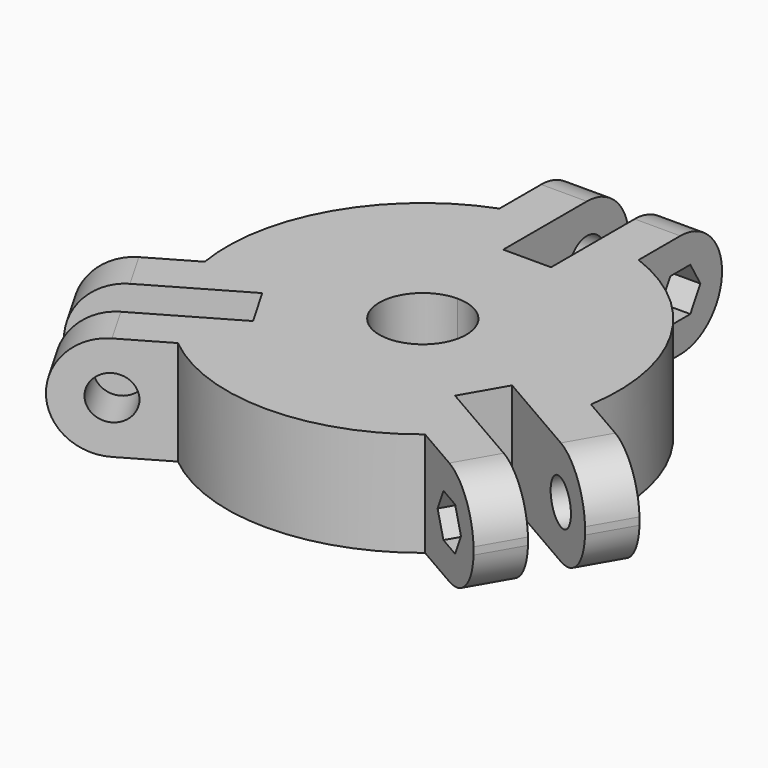
from build123d import *

# Parameters (mm, degrees)
F1_DEPTH  = 12
F3_DEPTH  = 25
F5_DEPTH  = 25
F7_DEPTH  = 25
F8_R      = 2.5
F9_DEPTH  = 5.6
F11_DEPTH = 7
F12_R     = 2.5
F13_DEPTH = 7
F15_DEPTH = 7
F16_R     = 2.5
F17_DEPTH = 7
F19_DEPTH = 7


with BuildPart() as f1:
    # F0 (on Top) → F1 (new body)
    with BuildSketch(Plane.XY):
        with BuildLine():
            ThreePointArc((0, 5), (3.5355339059, 3.5355339059), (5, 0))
            ThreePointArc((5, 0), (4.8296291314, -1.2940952255), (4.3301270189, -2.5))
            Line((4.3301270189, -2.5), (12.9903810568, -7.5))
            Line((12.9903810568, -7.5), (14.3653810568, -5.1184301396))
            Line((14.3653810568, -5.1184301396), (29.9538383249, -14.1184301396))
            Line((29.9538383249, -14.1184301396), (32.5788383249, -9.5717967697))
            Line((32.5788383249, -9.5717967697), (22.2122898066, -3.5866671921))
            ThreePointArc((22.2122898066, -3.5866671921), (19.4855715851, 11.25), (8, 21.0297408448))
            Line((8, 21.0297408448), (8, 33))
            Line((8, 33), (2.75, 33))
            Line((2.75, 33), (2.75, 15))
            Line((2.75, 15), (0, 15))
            Line((0, 15), (0, 5))
        make_face()
        with BuildLine():
            ThreePointArc((-4.3301270189, -2.5), (-4.3301270189, 2.5), (0, 5))
            Line((0, 5), (0, 15))
            Line((0, 15), (-2.75, 15))
            Line((-2.75, 15), (-2.75, 33))
            Line((-2.75, 33), (-8, 33))
            Line((-8, 33), (-8, 21.0297408448))
            ThreePointArc((-8, 21.0297408448), (-19.4855715851, 11.25), (-22.2122898066, -3.5866671921))
            Line((-22.2122898066, -3.5866671921), (-32.5788383249, -9.5717967697))
            Line((-32.5788383249, -9.5717967697), (-29.9538383249, -14.1184301396))
            Line((-29.9538383249, -14.1184301396), (-14.3653810568, -5.1184301396))
            Line((-14.3653810568, -5.1184301396), (-12.9903810568, -7.5))
            Line((-12.9903810568, -7.5), (-4.3301270189, -2.5))
        make_face()
        with BuildLine():
            Line((12.9903810568, -7.5), (4.3301270189, -2.5))
            ThreePointArc((4.3301270189, -2.5), (0, -5), (-4.3301270189, -2.5))
            Line((-4.3301270189, -2.5), (-12.9903810568, -7.5))
            Line((-12.9903810568, -7.5), (-11.6153810568, -9.8815698604))
            Line((-11.6153810568, -9.8815698604), (-27.2038383249, -18.8815698604))
            Line((-27.2038383249, -18.8815698604), (-24.5788383249, -23.4282032303))
            Line((-24.5788383249, -23.4282032303), (-14.2122898066, -17.4430736527))
            ThreePointArc((-14.2122898066, -17.4430736527), (0, -22.5), (14.2122898066, -17.4430736527))
            Line((14.2122898066, -17.4430736527), (24.5788383249, -23.4282032303))
            Line((24.5788383249, -23.4282032303), (27.2038383249, -18.8815698604))
            Line((27.2038383249, -18.8815698604), (11.6153810568, -9.8815698604))
            Line((11.6153810568, -9.8815698604), (12.9903810568, -7.5))
        make_face()
    extrude(amount=F1_DEPTH)

    # F2 (on face) → F3 (cut)
    with BuildSketch(Plane(origin=(-8, 0, 0), x_dir=(0, -1, 0), z_dir=(-1, 0, 0))):
        with BuildLine():
            ThreePointArc((-27.0148704224, 0), (-31.1055308437, 1.6106381651), (-33, 5.5778342276))
            Line((-33, 5.5778342276), (-33, 0))
            Line((-33, 0), (-27.0148704224, 0))
        make_face()
        with BuildLine():
            Line((-33, 5.5778342276), (-33, 6.4221657724))
            ThreePointArc((-33, 6.4221657724), (-33.0148704224, 6), (-33, 5.5778342276))
        make_face()
        with BuildLine():
            ThreePointArc((-33, 6.4221657724), (-31.1055308437, 10.3893618349), (-27.0148704224, 12))
            Line((-27.0148704224, 12), (-33, 12))
            Line((-33, 12), (-33, 6.4221657724))
        make_face()
    extrude(amount=-F3_DEPTH, mode=Mode.SUBTRACT)

    # F4 (on face) → F5 (cut)
    with BuildSketch(Plane(origin=(-4, 6.9282032303, 0), x_dir=(-0.8660254038, -0.5, 0), z_dir=(-0.5, 0.8660254038, 0))):
        with BuildLine():
            Line((33, 12), (27.0148704224, 12))
            ThreePointArc((27.0148704224, 12), (31.1055308437, 10.3893618349), (33, 6.4221657724))
            Line((33, 6.4221657724), (33, 12))
        make_face()
        with BuildLine():
            Line((33, 0), (33, 5.5778342276))
            ThreePointArc((33, 5.5778342276), (31.1055308437, 1.6106381651), (27.0148704224, 0))
            Line((27.0148704224, 0), (33, 0))
        make_face()
        with BuildLine():
            ThreePointArc((33, 5.5778342276), (33.0148704224, 6), (33, 6.4221657724))
            Line((33, 6.4221657724), (33, 5.5778342276))
        make_face()
    extrude(amount=-F5_DEPTH, mode=Mode.SUBTRACT)

    # F6 (on face) → F7 (cut)
    with BuildSketch(Plane(origin=(-4, -6.9282032303, 0), x_dir=(0.8660254038, -0.5, 0), z_dir=(-0.5, -0.8660254038, 0))):
        with BuildLine():
            Line((33, 12), (27.0148704224, 12))
            ThreePointArc((27.0148704224, 12), (31.1055308437, 10.3893618349), (33, 6.4221657724))
            Line((33, 6.4221657724), (33, 12))
        make_face()
        with BuildLine():
            Line((33, 0), (33, 5.5778342276))
            ThreePointArc((33, 5.5778342276), (31.1055308437, 1.6106381651), (27.0148704224, 0))
            Line((27.0148704224, 0), (33, 0))
        make_face()
        with BuildLine():
            ThreePointArc((33, 5.5778342276), (33.0148704224, 6), (33, 6.4221657724))
            Line((33, 6.4221657724), (33, 5.5778342276))
        make_face()
    extrude(amount=-F7_DEPTH, mode=Mode.SUBTRACT)

    # F8 (on face) → F9 (cut)
    with BuildSketch(Plane(origin=(4, -6.9282032303, 0), x_dir=(0.8660254038, 0.5, 0), z_dir=(0.5, -0.8660254038, 0))):
        with Locations((-27.0148704224, 6)):
            Circle(F8_R)
    extrude(amount=-F9_DEPTH, mode=Mode.SUBTRACT)

    # F10 (on face) → F11 (cut)
    with BuildSketch(Plane(origin=(-4, 6.9282032303, 0), x_dir=(-0.8660254038, -0.5, 0), z_dir=(-0.5, 0.8660254038, 0))):
        Polygon((28.4582460954, 8.5), (25.5714947494, 8.5), (24.1281190765, 6), (25.5714947494, 3.5), (28.4582460954, 3.5), (29.9016217684, 6), align=None)
    extrude(amount=-F11_DEPTH, mode=Mode.SUBTRACT)

    # F12 (on face) → F13 (cut)
    with BuildSketch(Plane(origin=(-8, 0, 0), x_dir=(0, -1, 0), z_dir=(-1, 0, 0))):
        with Locations((-27.0148704224, 6)):
            Circle(F12_R)
    extrude(amount=-F13_DEPTH, mode=Mode.SUBTRACT)

    # F14 (on face) → F15 (cut)
    with BuildSketch(Plane.YZ.offset(8)):
        Polygon((28.4582460954, 8.5), (25.5714947494, 8.5), (24.1281190765, 6), (25.5714947494, 3.5), (28.4582460954, 3.5), (29.9016217684, 6), align=None)
    extrude(amount=-F15_DEPTH, mode=Mode.SUBTRACT)

    # F16 (on face) → F17 (cut)
    with BuildSketch(Plane(origin=(4, 6.9282032303, 0), x_dir=(-0.8660254038, 0.5, 0), z_dir=(0.5, 0.8660254038, 0))):
        with Locations((-27.0148704224, 6)):
            Circle(F16_R)
    extrude(amount=-F17_DEPTH, mode=Mode.SUBTRACT)

    # F18 (on face) → F19 (cut)
    with BuildSketch(Plane(origin=(-4, -6.9282032303, 0), x_dir=(0.8660254038, -0.5, 0), z_dir=(-0.5, -0.8660254038, 0))):
        Polygon((28.4582460954, 8.5), (25.5714947494, 8.5), (24.1281190765, 6), (25.5714947494, 3.5), (28.4582460954, 3.5), (29.9016217684, 6), align=None)
    extrude(amount=-F19_DEPTH, mode=Mode.SUBTRACT)


solid = f1.part
